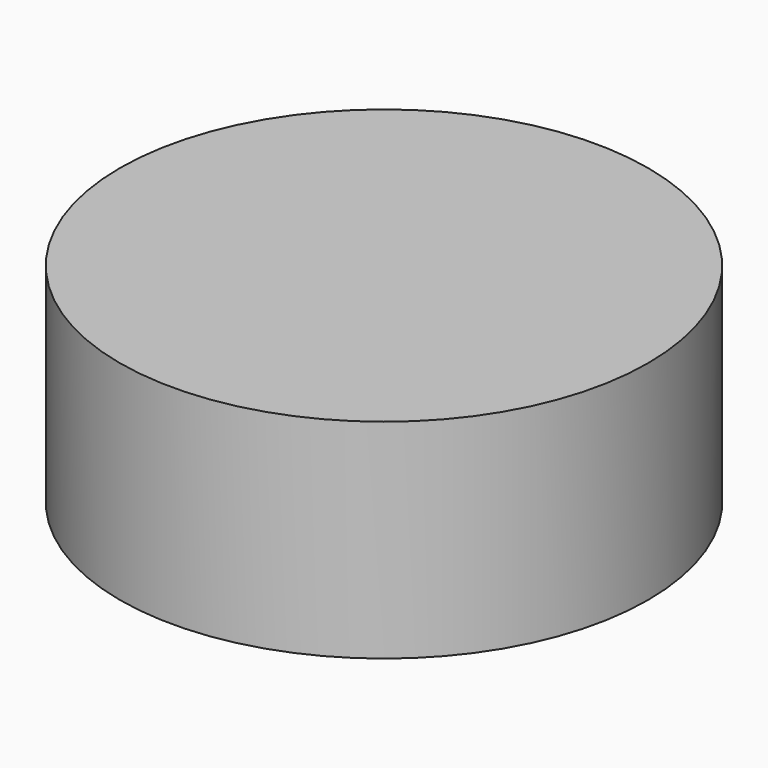
from build123d import *

# Parameters (mm, degrees)
F0_R     = 38
F1_DEPTH = 30


# Not quite as in the source:
# - a feature names something its author has since deleted; it is built from what else it names


with BuildPart() as f1:
    # F0 (on Top) → F1 (new body)
    with BuildSketch(Plane.XY):
        Circle(F0_R)
    extrude(amount=F1_DEPTH)


solid = f1.part
